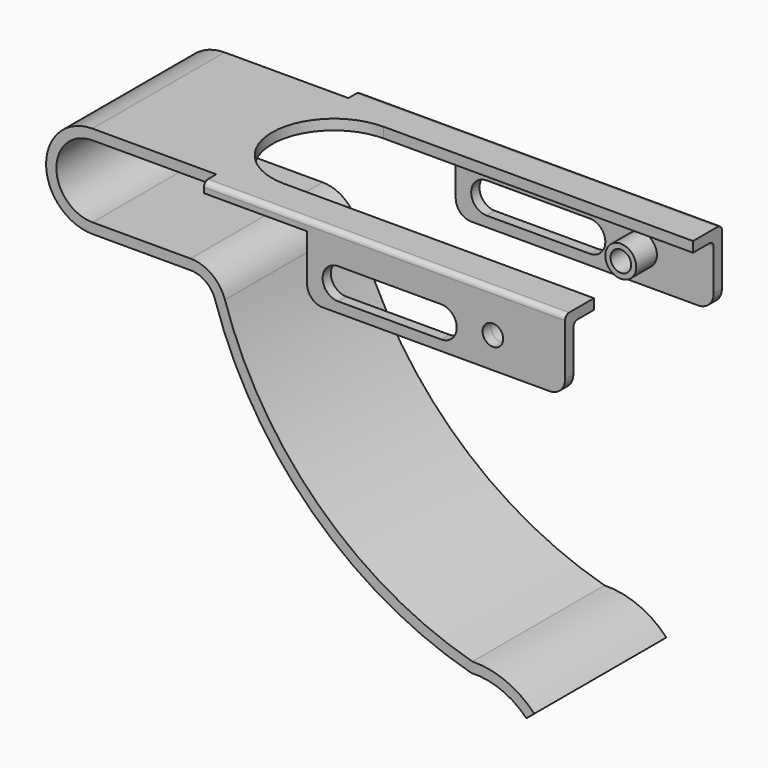
from build123d import *

# Parameters (mm, degrees)
F1_DEPTH  = 16
F2_W      = 70
F2_H      = 3
F3_DEPTH  = 2
F4_W      = 50
F4_H      = 14
F5_DEPTH  = 2
F6_R      = 1
F9_DEPTH  = 2
F11_DEPTH = 38.001
F13_D     = 4
F14_R     = 3
F14_R_2   = 2
F15_DEPTH = 5
F16_R     = 3


# Not quite as in the source:
# - a pattern or mirror of a feature is missing from the dataset's text; its kind, count and spacing are read off the source's solid


with BuildPart() as f1:
    # F0 (on Front) → F1 (new body)
    with BuildSketch(Plane.XZ):
        with BuildLine():
            Line((94, 9), (0, 9))
            ThreePointArc((0, 9), (-9, 0), (0, -9))
            Line((0, -9), (19, -9))
            ThreePointArc((19, -9), (21.9483530121, -9.9617807742), (23.7624383273, -12.4771141937))
            ThreePointArc((23.7624383273, -12.4771141937), (42.5404984663, -42.5461666629), (73.3918884835, -60.0091329916))
            ThreePointArc((73.3918884835, -60.0091329916), (79.2017940664, -60.9932244785), (84.0921252778, -64.2807919045))
            Line((84.0921252778, -64.2807919045), (85.6344375761, -63))
            ThreePointArc((85.6344375761, -63), (80.1625330731, -59.2251678092), (73.628769931, -58))
            ThreePointArc((73.628769931, -58), (43.8155502437, -40.9978046119), (25.6674136582, -11.8679598712))
            ThreePointArc((25.6674136582, -11.8679598712), (23.127694217, -8.3464930839), (19, -7))
            Line((19, -7), (0, -7))
            ThreePointArc((0, -7), (-7, 0), (0, 7))
            Line((0, 7), (94, 7))
            Line((94, 7), (94, 9))
        make_face()
    extrude(amount=F1_DEPTH)

    # F2 (on face) → F3 (join)
    with BuildSketch(Plane.XY.offset(9)):
        with Locations((59, -17.5)):
            Rectangle(F2_W, F2_H)
    extrude(amount=-F3_DEPTH)

    # F4 (on face) → F5 (join)
    with BuildSketch(Plane.XZ.offset(19)):
        with Locations((69, 2)):
            Rectangle(F4_W, F4_H)
    extrude(amount=-F5_DEPTH)

    # F6
    f6_edges = [f1.edges().sort_by_distance(p)[0] for p in [
        (69, -17, 7),
        (59, -19, 9),
    ]]
    fillet(f6_edges, radius=F6_R)

    # F7: F1 across plane


with BuildPart() as f1_1:
    add(f1.part)
    add(f1.part.mirror(Plane.XZ))

    # F8 (on face) → F9 (cut)
    with BuildSketch(Plane.XY.offset(9)):
        with BuildLine():
            Line((94, 12), (34, 12))
            ThreePointArc((34, 12), (22, 0), (34, -12))
            Line((34, -12), (94, -12))
            Line((94, -12), (94, 12))
        make_face()
    extrude(amount=-F9_DEPTH, mode=Mode.SUBTRACT)

    # F10 (on face) → F11 (cut, through all)
    with BuildSketch(Plane.XZ.offset(19)):
        with BuildLine():
            ThreePointArc((50, 3), (47, 0), (50, -3))
            Line((50, -3), (70, -3))
            ThreePointArc((70, -3), (73, 0), (70, 3))
            Line((70, 3), (50, 3))
        make_face()
    extrude(amount=-F11_DEPTH, mode=Mode.SUBTRACT)

    # F13 (through all)
    with Locations(Plane.XZ.offset(19)):
        with Locations((80, 1)):
            Hole(F13_D / 2)

    # F14 (on face) → F15 (join)
    with BuildSketch(Plane(origin=(0, -17, 0), x_dir=(-1, 0, 0), z_dir=(0, 1, 0))):
        with Locations((-80, 1)):
            Circle(F14_R)
        with Locations((-80, 1)):
            Circle(F14_R_2, mode=Mode.SUBTRACT)
    f15 = extrude(amount=F15_DEPTH)

    # F15_copies: F15 across plane
    add(f15.mirror(Plane.ZX))

    # F16
    f16_edges = [f1_1.edges().sort_by_distance(p)[0] for p in [
        (94, -18, -5),
        (94, 18, -5),
        (44, 18, -5),
        (44, -18, -5),
    ]]
    fillet(f16_edges, radius=F16_R)


solid = f1_1.part
